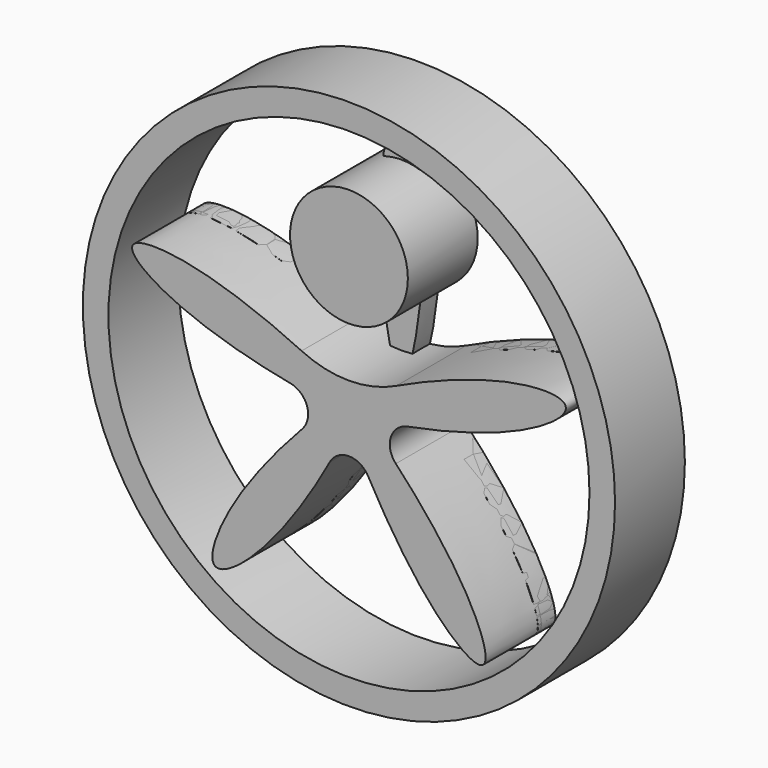
from build123d import *

# Parameters (mm, degrees)
F1_DEPTH = 6.35
F3_COUNT = 5
F5_DEPTH = 25.4
F4_R     = 17.1432552769
F4_R_2   = 77.4406377755
F4_R_3   = 69.9982637636


# Not quite as in the source:
# - the dataset's text gives a spline's control points without its knots; the knots are read off the source's solid


with BuildPart() as f1:
    # F0 (on Front) → F1 (new body)
    with BuildSketch(Plane.XZ):
        with BuildLine():
            add(Edge.make_bspline(
                [(0, 0), (1.1143386191, 3.4295816228), (-39.7623228402, 23.1971109266), (-71.4767096515, 23.2241907877), (-45.803314612, 4.6048500023), (-1.1143386191, -3.4295816228), (0, 0)],
                knots=[0, 0, 0, 0, 0.2922997589, 0.5, 0.7077002411, 1, 1, 1, 1], degree=3))
        make_face()
    extrude(amount=F1_DEPTH)


with BuildPart() as f3_1:
    # F3: instance of F1
    add(f1.part.rotate(Axis((0, -31.5394513309, 0), (0, -1, 0)), 1 * 360 / F3_COUNT))


with BuildPart() as f3_2:
    # F3: instance of F1
    add(f1.part.rotate(Axis((0, -31.5394513309, 0), (0, -1, 0)), 2 * 360 / F3_COUNT))


with BuildPart() as f3_3:
    # F3: instance of F1
    add(f1.part.rotate(Axis((0, -31.5394513309, 0), (0, -1, 0)), 3 * 360 / F3_COUNT))


with BuildPart() as f3_4:
    # F3: instance of F1
    add(f1.part.rotate(Axis((0, -31.5394513309, 0), (0, -1, 0)), 4 * 360 / F3_COUNT))


with BuildPart() as f5:
    # F4 (on Front) → F5 (new body)
    with BuildSketch(Plane.XZ):
        with BuildLine():
            ThreePointArc((13.7820680936, 9.675941025), (0, 6.5286873802), (-13.7820680936, 9.675941025))
            add(Edge.make_bspline(
                [(-13.7820680936, 9.675941025), (-21.725032175, 13.5032123812), (-46.4766068596, 23.2028440307), (-71.4767096515, 23.2241907877), (-51.2897707118, 8.5838405359), (-25.7197329357, 1.8992974565), (-17.0952302997, 0.3198876769)],
                knots=[0.149827914, 0.149827914, 0.149827914, 0.149827914, 0.2922997589, 0.5, 0.7077002411, 0.8487630367, 0.8487630367, 0.8487630367, 0.8487630367], degree=3))
            ThreePointArc((-17.0952302997, 0.3198876769), (-12.1998778517, -3.9639806057), (-13.6423065764, -10.3071188216))
            add(Edge.make_bspline(
                [(-13.6423065764, -10.3071188216), (-19.6913220011, -16.6542436322), (-36.4488412684, -37.0918436884), (-44.1750359687, -60.8017208434), (-24.013128264, -46.1269180522), (-9.7541737903, -23.8740044144), (-5.5869479449, -16.1596794457)],
                knots=[0.1512369633, 0.1512369633, 0.1512369633, 0.1512369633, 0.2922997589, 0.5, 0.7077002411, 0.8487630367, 0.8487630367, 0.8487630367, 0.8487630367], degree=3))
            ThreePointArc((-5.5869479449, -16.1596794457), (0, -12.8277107014), (5.5869479449, -16.1596794457))
            add(Edge.make_bspline(
                [(5.5869479449, -16.1596794457), (9.7541737903, -23.8740044144), (24.013128264, -46.1269180522), (44.1750359687, -60.8017208434), (36.4488412684, -37.0918436884), (19.6913220011, -16.6542436322), (13.6423065764, -10.3071188216)],
                knots=[0.1512369633, 0.1512369633, 0.1512369633, 0.1512369633, 0.2922997589, 0.5, 0.7077002411, 0.8487630367, 0.8487630367, 0.8487630367, 0.8487630367], degree=3))
            ThreePointArc((13.6423065764, -10.3071188216), (12.1998778517, -3.9639806057), (17.0952302997, 0.3198876769))
            add(Edge.make_bspline(
                [(17.0952302997, 0.3198876769), (25.7197329357, 1.8992974565), (51.2897707118, 8.5838405359), (71.4767096515, 23.2241907877), (46.4766068596, 23.2028440307), (21.725032175, 13.5032123812), (13.7820680936, 9.675941025)],
                knots=[0.1512369633, 0.1512369633, 0.1512369633, 0.1512369633, 0.2922997589, 0.5, 0.7077002411, 0.850172086, 0.850172086, 0.850172086, 0.850172086], degree=3))
        make_face()
    extrude(amount=F5_DEPTH)


with BuildPart() as f5b:
    # F4 (on Front) → F5, piece 2 (new body)
    with BuildSketch(Plane.XZ):
        with Locations((0, 38.2786873802)):
            Circle(F4_R)
    extrude(amount=F5_DEPTH)


with BuildPart() as f5c:
    # F4 (on Front) → F5, piece 3 (new body)
    with BuildSketch(Plane.XZ):
        with Locations((0, 0.516157012)):
            Circle(F4_R_2)
        with Locations((0, 0.516157012)):
            Circle(F4_R_3, mode=Mode.SUBTRACT)
    extrude(amount=F5_DEPTH)


solid = Compound([f1.part, f3_1.part, f3_2.part, f3_3.part, f3_4.part, f5.part, f5b.part, f5c.part])
